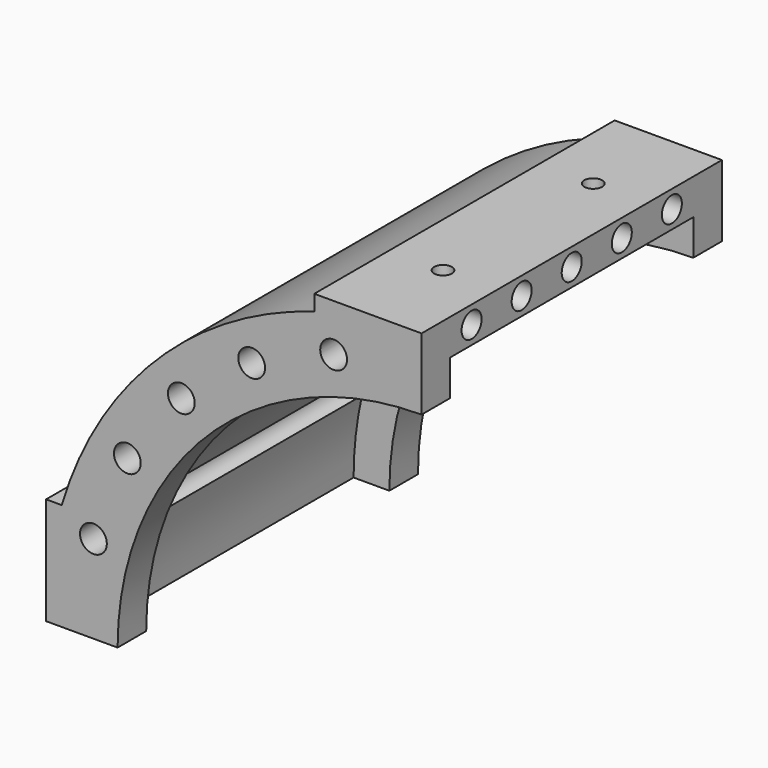
from build123d import *

# Parameters (mm, degrees)
F1_DEPTH  = 210
F2_W      = 210
F2_H      = 20
F3_DEPTH  = 60
F4_DEPTH  = 60
F5_R      = 7
F6_DEPTH  = 50
F8_D      = 15
F8_DEPTH  = 40
F8_TIP    = 4.5064546427
F10_DEPTH = 20
F12_DEPTH = 20
F14_D     = 15
F14_DEPTH = 220
F14_TIP   = 4.5064546427
F15_W     = 20
F15_H     = 15
F16_DEPTH = 200
F17_D     = 10
F17_DEPTH = 40
F17_TIP   = 3.0043030951
F18_R     = 7
F19_DEPTH = 50


# Not quite as in the source:
# - a feature names something its author has since deleted; it is built from what else it names


with BuildPart() as f1:
    # F0 (on Front) → F1 (new body)
    with BuildSketch(Plane.XZ):
        with BuildLine():
            Line((0, 190), (0, 210))
            ThreePointArc((0, 210), (-148.4924240492, 148.4924240492), (-210, 0))
            Line((-210, 0), (-190, 0))
            ThreePointArc((-190, 0), (-134.3502884254, 134.3502884254), (0, 190))
        make_face()
    extrude(amount=F1_DEPTH)

    # F2 (on face) → F3 (join)
    with BuildSketch(Plane.YZ):
        with Locations((-105, 200)):
            Rectangle(F2_W, F2_H)
    extrude(amount=-F3_DEPTH)

    # F4 (add): a face of the model
    f4_faces = [f1.faces().sort_by_distance(p)[0] for p in [
        (-200, -105, 0),
    ]]
    extrude(f4_faces, amount=-F4_DEPTH)

    # F5 (on face) → F6 (cut)
    with BuildSketch(Plane.YZ):
        with Locations((-175, 200)):
            Circle(F5_R)
        with Locations((-140, 200)):
            Circle(F5_R)
        with Locations((-105, 200)):
            Circle(F5_R)
        with Locations((-70, 200)):
            Circle(F5_R)
        with Locations((-35, 200)):
            Circle(F5_R)
    extrude(amount=-F6_DEPTH, mode=Mode.SUBTRACT)

    # F8
    with Locations(Plane.XY.offset(210)):
        with Locations((-30, -157.5), (-30, -52.5)):
            Hole(F8_D / 2, depth=F8_DEPTH)
            with Locations((0, 0, -(F8_DEPTH + F8_TIP / 2))):  # 118° drill point
                Cone(0, F8_D / 2, F8_TIP, mode=Mode.SUBTRACT)

    # F9 (on face) → F10 (join)
    with BuildSketch(Plane.XZ.offset(210)):
        with BuildLine():
            ThreePointArc((-170, 0), (-120.2081528017, 120.2081528017), (0, 170))
            Line((0, 170), (0, 190))
            ThreePointArc((0, 190), (-134.3502884254, 134.3502884254), (-190, 0))
            Line((-190, 0), (-170, 0))
        make_face()
    extrude(amount=-F10_DEPTH)

    # F11 (on face) → F12 (join)
    with BuildSketch(Plane(origin=(0, 0, 0), x_dir=(-1, 0, 0), z_dir=(0, 1, 0))):
        with BuildLine():
            ThreePointArc((0, 170), (120.2081528017, 120.2081528017), (170, 0))
            Line((170, 0), (190, 0))
            ThreePointArc((190, 0), (134.3502884254, 134.3502884254), (0, 190))
            Line((0, 190), (0, 170))
        make_face()
    extrude(amount=-F12_DEPTH)

    # F14
    with Locations(Plane.XZ.offset(210)):
        with Locations((-183.5259069949, 49.1756185695), (-164.544826719, 95), (-134.3502884254, 134.3502884254), (-95, 164.544826719), (-49.1756185695, 183.5259069949)):
            Hole(F14_D / 2, depth=F14_DEPTH)
            with Locations((0, 0, -(F14_DEPTH + F14_TIP / 2))):  # 118° drill point
                Cone(0, F14_D / 2, F14_TIP, mode=Mode.SUBTRACT)

    # F15 (on face) → F16 (join)
    with BuildSketch(Plane(origin=(0, 0, 0), x_dir=(-1, 0, 0), z_dir=(0, 1, 0))):
        with Locations((30, 202.5)):
            Rectangle(F15_W, F15_H)
    extrude(amount=-F16_DEPTH)

    # F17
    with Locations(Plane.XY.offset(210)):
        with Locations((-30, -52.5), (-30, -157.5)):
            Hole(F17_D / 2, depth=F17_DEPTH)
            with Locations((0, 0, -(F17_DEPTH + F17_TIP / 2))):  # 118° drill point
                Cone(0, F17_D / 2, F17_TIP, mode=Mode.SUBTRACT)

    # F18 (on face) → F19 (cut)
    with BuildSketch(Plane(origin=(0, 0, 0), x_dir=(1, 0, 0), z_dir=(0, 0, -1))):
        with Locations((-200, 35)):
            Circle(F18_R)
        with Locations((-200, 70)):
            Circle(F18_R)
        with Locations((-200, 105)):
            Circle(F18_R)
        with Locations((-200, 140)):
            Circle(F18_R)
        with Locations((-200, 175)):
            Circle(F18_R)
    extrude(amount=-F19_DEPTH, mode=Mode.SUBTRACT)


solid = f1.part
